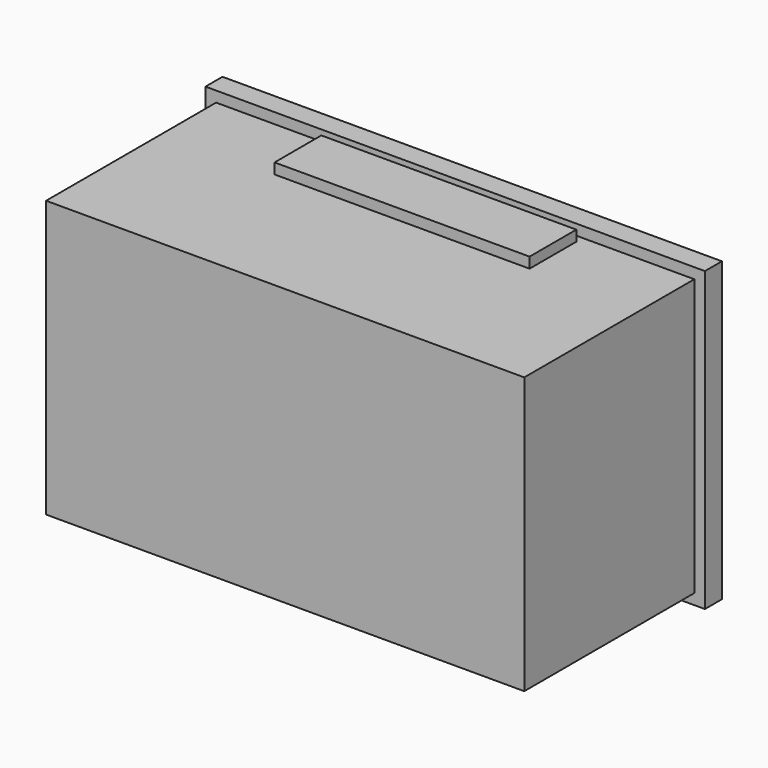
from build123d import *

# Parameters (mm, degrees)
F0_W     = 45
F0_H     = 26
F1_DEPTH = 22
F0_W_2   = 47
F0_H_2   = 28
F2_DEPTH = 2
F3_W     = 24
F3_H     = 5.5
F4_DEPTH = 1


# Not quite as in the source:
# - a pattern or mirror of a feature is missing from the dataset's text; its kind, count and spacing are read off the source's solid


with BuildPart() as f1:
    # F0 (on Front) → F1 (new body)
    with BuildSketch(Plane.XZ):
        Rectangle(F0_W, F0_H)
    extrude(amount=F1_DEPTH)

    # F0 (on Front) → F2 (join)
    with BuildSketch(Plane.XZ):
        Rectangle(F0_W_2, F0_H_2)
        Rectangle(F0_W, F0_H, mode=Mode.SUBTRACT)
    extrude(amount=F2_DEPTH)

    # F3 (on face) → F4 (join)
    with BuildSketch(Plane.XY.offset(13)):
        with Locations((0, -5.5)):
            Rectangle(F3_W, F3_H)
    f4 = extrude(amount=F4_DEPTH)

    # F4_copies: F4 across plane
    add(f4.mirror(Plane(origin=(0, 0, 0), x_dir=(-1, 0, 0), z_dir=(0, 0, -1))))


solid = f1.part
